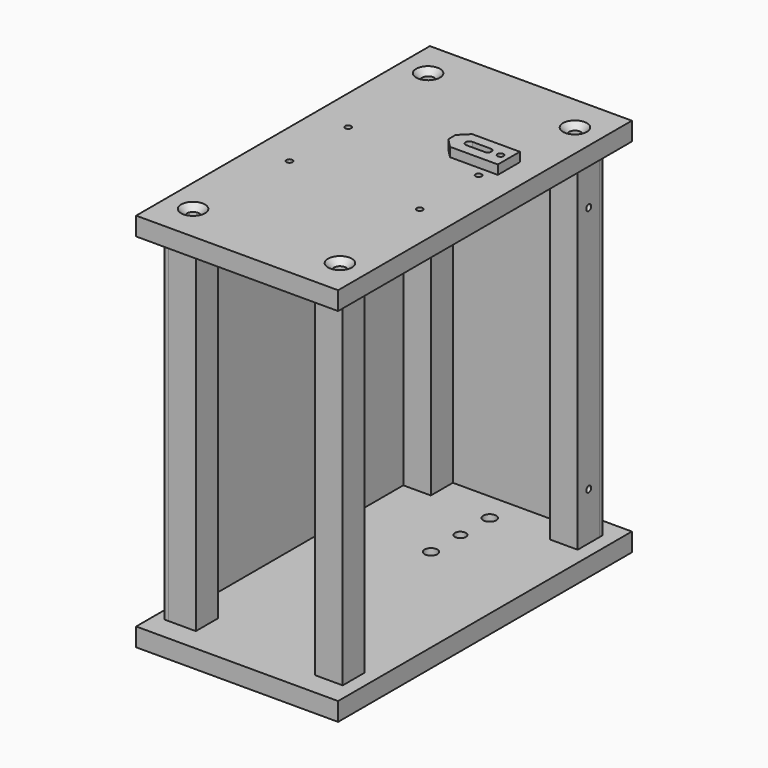
from build123d import *

# Parameters (mm, degrees)
F3_W            = 55
F3_H            = 200
F3_R            = 6.9331796816
F5_DEPTH        = 10
F6_D            = 6.6
F6_CSINK_D      = 13
F6_CSINK_ANGLE  = 90
F8_W            = 55
F8_H            = 200
F9_DEPTH        = 10
F11_D           = 6.6
F11_CSINK_D     = 13
F11_CSINK_ANGLE = 90
F13_W           = 15
F13_H           = 15
F14_DEPTH       = 187
F15_D           = 5
F15_DEPTH       = 12
F15_START       = 10
F15_TIP         = 1.5021515476
F16_D           = 5
F16_DEPTH       = 12
F16_START       = 10
F16_TIP         = 1.5021515476
F19_D           = 7
F20_D           = 6
F22_W           = 95
F22_H           = 187
F23_DEPTH       = 2
F26_D           = 3.3
F26_DEPTH       = 12
F26_TIP         = 0.9914200214
F27_D           = 3.3
F27_DEPTH       = 12
F27_TIP         = 0.9914200214
F28_D           = 4.5
F30_W           = 31
F30_H           = 15
F31_DEPTH       = 5
F32_SIZE        = 5
F34_DEPTH       = 5
F35_D           = 3.3
F36_D           = 3.3
F37_W           = 175
F37_H           = 187
F38_DEPTH       = 2
F39_D           = 4.5
F40_R           = 15
F41_DEPTH       = 4
F42_R           = 10
F43_DEPTH       = 1


# Not quite as in the source:
# - a pattern or mirror of a feature is missing from the dataset's text; its kind, count and spacing are read off the source's solid


with BuildPart() as f5:
    # F3 (on Top) → F5 (new body)
    with BuildSketch(Plane.XY):
        with Locations((27.5, -52)):
            Rectangle(F3_W, F3_H)
        with Locations((40, -132)):
            Circle(F3_R, mode=Mode.SUBTRACT)
        with Locations((40, 28)):
            Circle(F3_R, mode=Mode.SUBTRACT)
        with Locations((40, -132)):
            Circle(F3_R)
        with Locations((40, 28)):
            Circle(F3_R)
    extrude(amount=F5_DEPTH)

    # F6 (through all)
    with Locations(Plane(origin=(0, 0, 0), x_dir=(1, 0, 0), z_dir=(0, 0, -1))):
        with Locations((40, -28), (40, 132)):
            CounterSinkHole(F6_D / 2, F6_CSINK_D / 2, counter_sink_angle=F6_CSINK_ANGLE)

    # F7: F5 across plane


with BuildPart() as f5_1:
    add(f5.part)
    add(f5.part.mirror(Plane.YZ))

    # F19 (through all)
    with Locations(Plane(origin=(0, 0, 0), x_dir=(1, 0, 0), z_dir=(0, 0, -1))):
        with Locations((0, -20), (0, 20)):
            Hole(F19_D / 2)

    # F20 (through all)
    with Locations(Plane(origin=(0, 0, 0), x_dir=(1, 0, 0), z_dir=(0, 0, -1))):
        with Locations((0, 0)):
            Hole(F20_D / 2)


with BuildPart() as f9:
    # F8 (on offset) → F9 (new body)
    with BuildSketch(Plane.XY.offset(197)):
        with Locations((27.5, -52)):
            Rectangle(F8_W, F8_H)
    extrude(amount=F9_DEPTH)

    # F11 (through all)
    with Locations(Plane.XY.offset(207)):
        with Locations((40, 28), (40, -132)):
            CounterSinkHole(F11_D / 2, F11_CSINK_D / 2, counter_sink_angle=F11_CSINK_ANGLE)

    # F12: F9 across plane


with BuildPart() as f9_1:
    add(f9.part)
    add(f9.part.mirror(Plane.YZ))

    # F36 (through all)
    with Locations(Plane.XY.offset(215.6)):
        with Locations((35.5, -32), (35.5, -72)):
            f36 = Hole(F36_D / 2)

    # F36_copies: F36 across plane
    add(f36.mirror(Plane(origin=(0, 0, 0), x_dir=(0, 0, -1), z_dir=(-1, 0, 0))), mode=Mode.SUBTRACT)


with BuildPart() as f14:
    # F13 (on face) → F14 (new body, through all)
    with BuildSketch(Plane.XY.offset(10)):
        with Locations((40, 28)):
            Rectangle(F13_W, F13_H)
    extrude(amount=F14_DEPTH)

    # F15
    # its depths count from where the whole tool has entered the part; down to there all is cleared
    with Locations(Plane(origin=(0, 0, 0), x_dir=(1, 0, 0), z_dir=(0, 0, -1)).offset(-F15_START)):
        with Locations((40, -28)):
            Hole(F15_D / 2, depth=F15_DEPTH)
            with Locations((0, 0, -(F15_DEPTH + F15_TIP / 2))):  # 118° drill point
                Cone(0, F15_D / 2, F15_TIP, mode=Mode.SUBTRACT)

    # F16
    # its depths count from where the whole tool has entered the part; down to there all is cleared
    with Locations(Plane.XY.offset(207).offset(-F16_START)):
        with Locations((40, 28)):
            Hole(F16_D / 2, depth=F16_DEPTH)
            with Locations((0, 0, -(F16_DEPTH + F16_TIP / 2))):  # 118° drill point
                Cone(0, F16_D / 2, F16_TIP, mode=Mode.SUBTRACT)


with BuildPart() as f17_1:
    # F17: instance of F14
    add(f14.part.mirror(Plane(origin=(55, -52, 0), x_dir=(1, 0, 0), z_dir=(0, -1, 0))))


with BuildPart() as f18_1:
    # F18: instance of F17_1
    add(f17_1.part.mirror(Plane.YZ))


with BuildPart() as f18_2:
    # F18: instance of F14
    add(f14.part.mirror(Plane.YZ))


with BuildPart() as f23:
    # F22 (on face) → F23 (new body)
    with BuildSketch(Plane(origin=(0, 35.5, 0), x_dir=(-1, 0, 0), z_dir=(0, 1, 0))):
        with Locations((0, 103.5)):
            Rectangle(F22_W, F22_H)
    extrude(amount=F23_DEPTH)

    # F28 (through all)
    with Locations(Plane(origin=(0, 35.5, 0), x_dir=(-1, 0, 0), z_dir=(0, -1, 0))):
        with Locations((-40, -179), (-40, -28)):
            f28 = Hole(F28_D / 2)

    # F28_copies: F28 across plane
    add(f28.mirror(Plane(origin=(0, 0, 0), x_dir=(0, 0, -1), z_dir=(-1, 0, 0))), mode=Mode.SUBTRACT)


with BuildPart() as f14_1:
    add(f14.part)

    # F26
    with Locations(Plane(origin=(0, 35.5, 0), x_dir=(-1, 0, 0), z_dir=(0, 1, 0))):
        with Locations((-40, 179), (-40, 28)):
            Hole(F26_D / 2, depth=F26_DEPTH)
            with Locations((0, 0, -(F26_DEPTH + F26_TIP / 2))):  # 118° drill point
                Cone(0, F26_D / 2, F26_TIP, mode=Mode.SUBTRACT)

    # F27
    with Locations(Plane.YZ.offset(47.5)):
        with Locations((28, 171), (28, 36)):
            Hole(F27_D / 2, depth=F27_DEPTH)
            with Locations((0, 0, -(F27_DEPTH + F27_TIP / 2))):  # 118° drill point
                Cone(0, F27_D / 2, F27_TIP, mode=Mode.SUBTRACT)


with BuildPart() as f31:
    # F30 (on offset) → F31 (new body)
    with BuildSketch(Plane.XY.offset(215.6)):
        with Locations((36.5, -32)):
            Rectangle(F30_W, F30_H)
    extrude(amount=F31_DEPTH)

    # F32
    f32_edges = [f31.edges().sort_by_distance(p)[0] for p in [
        (21, -39.5, 218.1),
        (21, -24.5, 218.1),
    ]]
    chamfer(f32_edges, length=F32_SIZE)

    # F33 (on face) → F34 (cut, through all)
    with BuildSketch(Plane.XY.offset(220.6)):
        with BuildLine():
            ThreePointArc((30.5, -30), (28.5, -32), (30.5, -34))
            Line((30.5, -34), (40.5, -34))
            ThreePointArc((40.5, -34), (42.5, -32), (40.5, -30))
            Line((40.5, -30), (30.5, -30))
        make_face()
    extrude(amount=-F34_DEPTH, mode=Mode.SUBTRACT)

    # F35 (through all)
    with Locations(Plane(origin=(0, 0, 215.6), x_dir=(1, 0, 0), z_dir=(0, 0, -1))):
        with Locations((47.5, 32)):
            Hole(F35_D / 2)


with BuildPart() as f38:
    # F37 (on face) → F38 (new body)
    with BuildSketch(Plane(origin=(-47.5, 0, 0), x_dir=(0, -1, 0), z_dir=(-1, 0, 0))):
        with Locations((52, 103.5)):
            Rectangle(F37_W, F37_H)
    extrude(amount=F38_DEPTH)

    # F39 (through all)
    with Locations(Plane.YZ.offset(47.5)):
        with Locations((-132, 171), (-132, 36), (28, 36), (28, 171)):
            Hole(F39_D / 2)


with BuildPart() as f41:
    # F40 (on face) → F41 (new body)
    with BuildSketch(Plane(origin=(0, 0, 0), x_dir=(1, 0, 0), z_dir=(0, 0, -1))):
        Circle(F40_R)
    extrude(amount=F41_DEPTH)

    # F42 (on face) → F43 (join)
    with BuildSketch(Plane(origin=(0, 0, -4), x_dir=(1, 0, 0), z_dir=(0, 0, -1))):
        Circle(F42_R)
    extrude(amount=F43_DEPTH)


solid = Compound([f5_1.part, f9_1.part, f17_1.part, f18_1.part, f18_2.part, f23.part, f14_1.part, f31.part, f38.part, f41.part])
